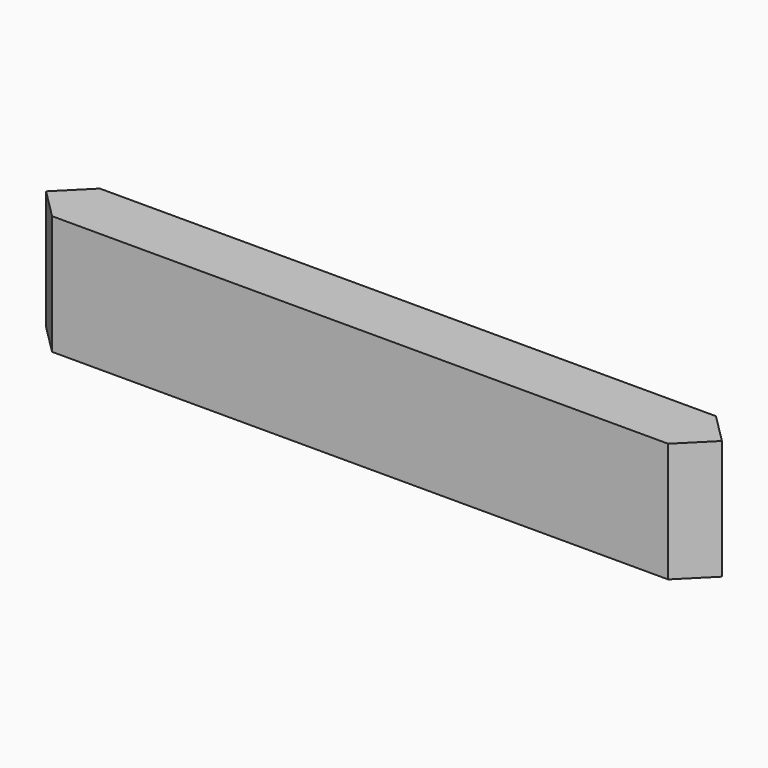
from build123d import *

# Parameters (mm, degrees)
F0_W             = 6.35
F0_H             = 12.7
F1_DEPTH         = 35.92068
F3_DEPTH         = 6.351
F3_DEPTH_BACK    = 6.351
F3_COPIES2_COUNT = 2


# Not quite as in the source:
# - a pattern or mirror of a feature is missing from the dataset's text; its kind, count and spacing are read off the source's solid


with BuildPart() as f1:
    # F0 (on Right) → F1 (new body, symmetric)
    with BuildSketch(Plane.YZ):
        Rectangle(F0_W, F0_H)
    extrude(amount=F1_DEPTH, both=True)

    # F2 (on Top) → F3 (cut, two sides)
    with BuildSketch(Plane.XY) as f3_sk:
        Polygon((-35.92068, 3.175), (-35.92068, 0), (-32.74568, 3.175), align=None)
    f3 = extrude(amount=-F3_DEPTH, mode=Mode.SUBTRACT) + extrude(f3_sk.sketch, amount=F3_DEPTH_BACK, mode=Mode.SUBTRACT)

    # F3_copies: F3 across plane
    add(f3.mirror(Plane(origin=(0, 0, 0), x_dir=(0, 0, -1), z_dir=(0, -1, 0))), mode=Mode.SUBTRACT)

    # F3_copies1: F3 across plane
    add(f3.mirror(Plane(origin=(0, 0, 0), x_dir=(0, 0, 1), z_dir=(1, 0, 0))), mode=Mode.SUBTRACT)

    # F3_copies2: F3 ×2 about axis
    f3_copies2_axis = Axis((0, 0, 0), (0, 0, 1))
    for i in range(1, F3_COPIES2_COUNT):
        add(f3.rotate(f3_copies2_axis, i * 360 / F3_COPIES2_COUNT), mode=Mode.SUBTRACT)


solid = f1.part
